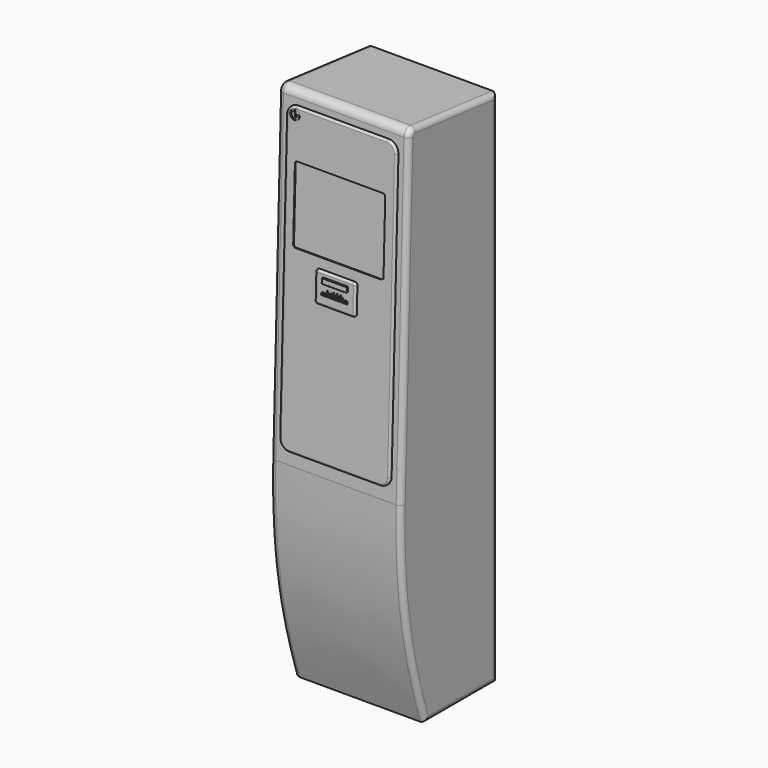
from build123d import *

# Parameters (mm, degrees)
F1_DEPTH     = 330.2
F3_DEPTH     = 6.35
F4_R         = 5.08
F6_DEPTH     = 2.54
F7_DEPTH     = 6.35
F8_R         = 5.08
F9_W         = 63.5
F9_H         = 6.35
F9_W_2       = 61.5422427654
F9_H_2       = 4.4705867767
F10_DEPTH    = 5.08
F11_T1_DEPTH = 88.9
F12_W        = 5.4762065411
F12_H        = 5.4786801338
F12_W_2      = 5.9325397015
F12_W_3      = 5.7043433189
F12_H_2      = 5.707025528
F12_W_4      = 5.4761767387
F12_H_3      = 5.4787397385
F12_W_5      = 6.1607062817
F13_DEPTH    = 1.27
F14_R        = 12.2001792315
F14_R_2      = 1.4877319336
F15_DEPTH    = 1.27
F17_DEPTH    = 3.81
F18_R        = 1.27
F19_R        = 12.7
F20_R        = 12.7


# Not quite as in the source:
# - a fillet or chamfer that OpenCascade refuses, or shapes differently, is made with other operations: its cross-section is extruded or revolved along the edge and cut away or added
# - ends of sketch curves that miss each other by under 0.0002 mm in the source are joined


with BuildPart() as f1:
    # F0 (on Right) → F1 (new body)
    with BuildSketch(Plane.YZ):
        with BuildLine():
            Line((-38.1692965456, -816.6212190319), (190.4307034544, -816.6212190319))
            Line((190.4307034544, -816.6212190319), (190.3661012281, -308.6212231396))
            Line((190.3661012281, -308.6212231396), (190.2637533991, 496.1915463583))
            Line((190.2637533991, 496.1915463583), (-68.5663730615, 524.558862898))
            ThreePointArc((-68.5663730615, 524.558862898), (-83.1393453573, 519.9997939801), (-89.6829224344, 506.2034817928))
            Line((-89.6829224344, 506.2034817928), (-114.3673987619, -302.4652168628))
            ThreePointArc((-114.3673987619, -302.4652168628), (-114.3683286205, -302.4963032721), (-114.3692204156, -302.5273907967))
            add(Edge.make_bspline(
                [(-114.3692204156, -302.5273907967), (-114.3698313563, -302.5482481048), (-114.3703658253, -302.5691068772), (-114.3708999527, -302.5899649767)],
                knots=[0, 0, 0, 0, 0.0503004337, 0.0503004337, 0.0503004337, 0.0503004337], degree=3))
            add(Edge.make_bspline(
                [(-114.3708999527, -302.5899649767), (-119.8890365614, -518.077613362), (-88.9373327837, -661.7395994869), (-38.1692965456, -816.6212190319)],
                knots=[0.0503004337, 0.0503004337, 0.0503004337, 0.0503004337, 519.7104063101, 519.7104063101, 519.7104063101, 519.7104063101], degree=3))
        make_face()
    extrude(amount=F1_DEPTH)

    # F2 (on face) → F3 (join)
    with BuildSketch(Plane(origin=(0, -105.0368290915, 3.2062315823), x_dir=(1, 0, 0), z_dir=(0, -0.9995344426, 0.0305106211))):
        with BuildLine():
            Line((279.2403237975, 487.7765979096), (50.6403237975, 487.7765979096))
            ThreePointArc((50.6403237975, 487.7765979096), (32.6798115554, 480.3371101518), (25.2403237975, 462.3765979096))
            Line((25.2403237975, 462.3765979096), (25.2403237975, -248.8234020904))
            ThreePointArc((25.2403237975, -248.8234020904), (32.6798115554, -266.7839143325), (50.6403237975, -274.2234020904))
            Line((50.6403237975, -274.2234020904), (279.2403237975, -274.2234020904))
            ThreePointArc((279.2403237975, -274.2234020904), (297.2008360397, -266.7839143325), (304.6403237975, -248.8234020904))
            Line((304.6403237975, -248.8234020904), (304.6403237975, 462.3765979096))
            ThreePointArc((304.6403237975, 462.3765979096), (297.2008360397, 480.3371101518), (279.2403237975, 487.7765979096))
        make_face()
    extrude(amount=F3_DEPTH)

    # F4
    f4_edges = [f1.edges().sort_by_distance(p)[0] for p in [
        (164.940324, -96.501506, 490.949484),
        (304.640324, -108.126052, 110.126861),
        (164.940324, -119.750599, -270.695761),
        (32.679812, -119.523616, -263.259737),
        (297.200836, -119.523616, -263.259737),
        (297.200836, -96.728489, 483.51346),
        (32.679812, -96.728489, 483.51346),
        (25.240324, -108.126052, 110.126861),
    ]]
    fillet(f4_edges, radius=F4_R)

    # F5 (on face) → F6 (cut)
    with BuildSketch(Plane(origin=(0, -111.3838728021, 3.3999740265), x_dir=(1, 0, 0), z_dir=(0, -0.9995344426, 0.0305106211))):
        with BuildLine():
            Line((272.2935825759, 368.3965979096), (56.3935825759, 368.3965979096))
            ThreePointArc((56.3935825759, 368.3965979096), (51.9034545153, 366.5367259702), (50.0435825759, 362.0465979096))
            Line((50.0435825759, 362.0465979096), (50.0435825759, 184.2465979096))
            ThreePointArc((50.0435825759, 184.2465979096), (51.9034545153, 179.7564698491), (56.3935825759, 177.8965979096))
            Line((56.3935825759, 177.8965979096), (272.2935825759, 177.8965979096))
            ThreePointArc((272.2935825759, 177.8965979096), (276.7837106364, 179.7564698491), (278.6435825759, 184.2465979096))
            Line((278.6435825759, 184.2465979096), (278.6435825759, 362.0465979096))
            ThreePointArc((278.6435825759, 362.0465979096), (276.7837106364, 366.5367259702), (272.2935825759, 368.3965979096))
        make_face()
    extrude(amount=-F6_DEPTH, mode=Mode.SUBTRACT)

    # F5 (on face) → F7 (join)
    with BuildSketch(Plane(origin=(0, -111.3838728021, 3.3999740265), x_dir=(1, 0, 0), z_dir=(0, -0.9995344426, 0.0305106211))):
        with BuildLine():
            Line((207.2245373726, 152.4965979096), (118.3245373726, 152.4965979096))
            ThreePointArc((118.3245373726, 152.4965979096), (113.8344093121, 150.6367259702), (111.9745373726, 146.1465979096))
            Line((111.9745373726, 146.1465979096), (111.9745373726, 82.6465979096))
            ThreePointArc((111.9745373726, 82.6465979096), (113.8344093121, 78.1564698491), (118.3245373726, 76.2965979096))
            Line((118.3245373726, 76.2965979096), (207.2245373726, 76.2965979096))
            ThreePointArc((207.2245373726, 76.2965979096), (211.7146654331, 78.1564698491), (213.5745373726, 82.6465979096))
            Line((213.5745373726, 82.6465979096), (213.5745373726, 146.1465979096))
            ThreePointArc((213.5745373726, 146.1465979096), (211.7146654331, 150.6367259702), (207.2245373726, 152.4965979096))
        make_face()
    extrude(amount=F7_DEPTH)

    # F8
    f8_edges = [f1.edges().sort_by_distance(p)[0] for p in [
        (162.774537, -113.078151, 156.019318),
        (113.834409, -113.134896, 154.160312),
        (111.974537, -114.240605, 117.937056),
        (113.834409, -115.346314, 81.7138),
        (162.774537, -115.40306, 79.854794),
        (211.714665, -115.346314, 81.7138),
        (213.574537, -114.240605, 117.937056),
        (211.714665, -113.134896, 154.160312),
    ]]
    fillet(f8_edges, radius=F8_R)

    # F9 (on face) → F10 (join)
    with BuildSketch(Plane(origin=(0, -117.7309165128, 3.5937164707), x_dir=(1, 0, 0), z_dir=(0, -0.9995344426, 0.0305106211))):
        with Locations((162.8764543798, 104.186504372)):
            Rectangle(F9_W, F9_H)
        with Locations((162.8231231239, 104.1027204593)):
            Rectangle(F9_W_2, F9_H_2, mode=Mode.SUBTRACT)
    extrude(amount=F10_DEPTH)

    # F11: fillet of radius 5.08 on 1 edges, made by hand

    # F11_s2 → F11_t1 (cut)
    with BuildSketch(Plane.YZ.offset(118.4264543798)):
        with BuildLine():
            ThreePointArc((-114.6489927728, 104.558194192), (-118.1940262129, 106.1549963188), (-119.5716337859, 109.7908231159))
            Line((-119.5716337859, 109.7908231159), (-119.7266277413, 104.7131881474))
            Line((-119.7266277413, 104.7131881474), (-114.6489927728, 104.558194192))
        make_face()
    extrude(amount=F11_T1_DEPTH, mode=Mode.SUBTRACT)

    # F12 (on face) → F13 (cut)
    with BuildSketch(Plane(origin=(0, -117.7309165128, 3.5937164707), x_dir=(1, 0, 0), z_dir=(0, -0.9995344426, 0.0305106211))):
        with Locations((144.8540896177, 112.5199238459)):
            Rectangle(F12_W, F12_H)
        with Locations((153.7528842688, 112.5199238459)):
            Rectangle(F12_W_2, F12_H)
        with Locations((162.3094439507, 112.8623227278)):
            Rectangle(F12_W_3, F12_H_2)
        with Locations((170.8659887314, 112.9764656226)):
            Rectangle(F12_W_4, F12_H_3)
        with Locations((179.4225484133, 112.8623227278)):
            Rectangle(F12_W_5, F12_H_2)
    extrude(amount=-F13_DEPTH, mode=Mode.SUBTRACT)

    # F14 (on face) → F15 (cut)
    with BuildSketch(Plane(origin=(0, -111.3838728021, 3.3999740265), x_dir=(1, 0, 0), z_dir=(0, -0.9995344426, 0.0305106211))):
        with Locations((47.6859843219, 468.5862184885)):
            Circle(F14_R)
        with BuildLine():
            ThreePointArc((59.2139227797, 468.5862184885), (40.2083352892, 460.4597679651), (47.6859843219, 479.7298566756))
            Line((47.6859843219, 479.7298566756), (47.6859843219, 479.0266872767))
            ThreePointArc((47.6859843219, 479.0266872767), (40.8408683265, 461.3953089073), (58.3340651638, 468.5862184885))
            Line((58.3340651638, 468.5862184885), (48.8012617315, 468.5862184885))
            Line((48.8012617315, 468.5862184885), (48.8012617315, 469.2769171122))
            Line((48.8012617315, 469.2769171122), (59.1431124617, 469.2769171122))
            Line((59.1431124617, 469.2769171122), (59.2139227797, 468.5862184885))
        make_face(mode=Mode.SUBTRACT)
        with Locations((43.3804055537, 474.8469711664)):
            Circle(F14_R_2, mode=Mode.SUBTRACT)
        Polygon((46.747740158, 462.8656031016), (46.747740158, 476.3347031), (47.7390957857, 476.3347031), (47.7390957857, 463.9282347086), (51.2404328073, 463.9282347086), (51.2404328073, 462.8656031016), align=None, mode=Mode.SUBTRACT)
    extrude(amount=-F15_DEPTH, mode=Mode.SUBTRACT)

    # F16 (on face) → F17 (join)
    with BuildSketch(Plane(origin=(0, -117.7309165128, 3.5937164707), x_dir=(1, 0, 0), z_dir=(0, -0.9995344426, 0.0305106211))):
        with BuildLine():
            ThreePointArc((131.1264543798, 127.8425344419), (131.4984287677, 126.9445088298), (132.3964543798, 126.5725344419))
            Line((132.3964543798, 126.5725344419), (193.3564543798, 126.5725344419))
            ThreePointArc((193.3564543798, 126.5725344419), (194.2544799919, 126.9445088298), (194.6264543798, 127.8425344419))
            Line((194.6264543798, 127.8425344419), (194.6264543798, 138.8177083969))
            ThreePointArc((194.6264543798, 138.8177083969), (194.2544799919, 139.715734009), (193.3564543798, 140.0877083969))
            Line((193.3564543798, 140.0877083969), (132.3964543798, 140.0877083969))
            ThreePointArc((132.3964543798, 140.0877083969), (131.4984287677, 139.715734009), (131.1264543798, 138.8177083969))
            Line((131.1264543798, 138.8177083969), (131.1264543798, 127.8425344419))
        make_face()
    extrude(amount=F17_DEPTH)

    # F18
    f18_edges = [f1.edges().sort_by_distance(p)[0] for p in [
        (194.626454, -117.471158, 136.978011),
    ]]
    fillet(f18_edges, radius=F18_R)

    # F19
    f19_edges = [f1.edges().sort_by_distance(p)[0] for p in [
        (330.2, 76.130703, -816.621219),
        (330.2, 190.347228, -160.214836),
        (330.2, 60.84869, 510.375205),
        (330.2, -83.139345, 519.999794),
        (330.2, -102.025161, 101.869132),
        (330.2, -114.368329, -302.496303),
        (330.2, -114.370089, -302.558677),
        (330.2, -100.348944, -563.178218),
    ]]
    fillet(f19_edges, radius=F19_R)

    # F20
    f20_edges = [f1.edges().sort_by_distance(p)[0] for p in [
        (0, 76.130703, -816.621219),
        (0, 190.347228, -160.214836),
        (0, 60.84869, 510.375205),
        (0, -83.139345, 519.999794),
        (0, -102.025161, 101.869132),
        (0, -114.368329, -302.496303),
        (0, -114.370089, -302.558677),
        (0, -100.348944, -563.178218),
    ]]
    fillet(f20_edges, radius=F20_R)


solid = f1.part
